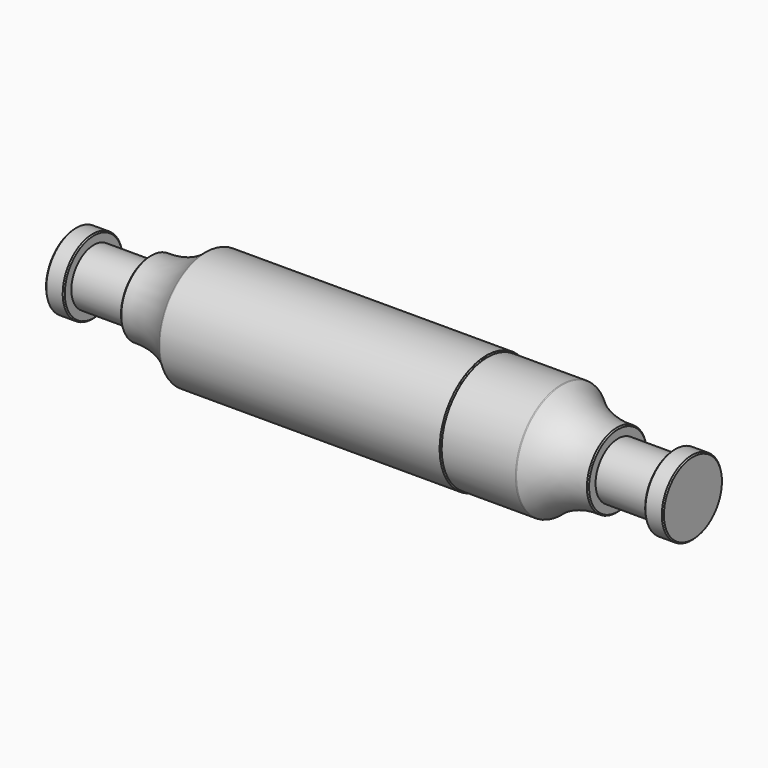
from build123d import *


# Not quite as in the source:
# - a fillet or chamfer that OpenCascade refuses, or shapes differently, is made with other operations: its cross-section is extruded or revolved along the edge and cut away or added


with BuildPart() as f1:
    # F0 (on Front) → F1 (revolve)
    with BuildSketch(Plane.XZ):
        with BuildLine():
            Line((-447.1154779911, 50.8), (-447.1154779911, 0))
            Line((-447.1154779911, 0), (391.0845220089, 0))
            Line((391.0845220089, 0), (391.0845220089, 50.8))
            Line((391.0845220089, 50.8), (365.6845220089, 50.8))
            Line((365.6845220089, 50.8), (365.6845220089, 38.1))
            Line((365.6845220089, 38.1), (289.4845220089, 38.1))
            Line((289.4845220089, 38.1), (289.4845220089, 50.8))
            ThreePointArc((289.4845220089, 50.8), (248.5849137461, 56.3889737285), (213.2845220089, 77.7875))
            Line((213.2845220089, 77.7875), (111.6845220089, 77.7875))
            Line((111.6845220089, 77.7875), (111.6845220089, 79.375))
            Line((111.6845220089, 79.375), (-269.3154779911, 79.375))
            ThreePointArc((-269.3154779911, 79.375), (-304.4294339656, 57.1247159319), (-345.5154779911, 50.8))
            Line((-345.5154779911, 50.8), (-345.5154779911, 38.1))
            Line((-345.5154779911, 38.1), (-421.7154779911, 38.1))
            Line((-421.7154779911, 38.1), (-421.7154779911, 50.8))
            Line((-421.7154779911, 50.8), (-447.1154779911, 50.8))
        make_face()
    revolve(axis=Axis((-28.0154779911, 0, 0), (1, 0, 0)))

    # F2: chamfer of 1.5875 on 8 edges, made by hand

    # F2_s1 → F2_t2 (revolve, cut)
    with BuildSketch(Plane.XZ):
        Polygon((-445.5279779911, 50.8), (-447.1154779911, 49.2125), (-447.1154779911, 50.8), align=None)
    revolve(axis=Axis((-447.1154779911, 0, 0), (1, 0, 0)), mode=Mode.SUBTRACT)

    # F2_s3 → F2_t4 (revolve, cut)
    with BuildSketch(Plane.XZ):
        Polygon((-421.7154779911, 49.2125), (-423.3029779911, 50.8), (-421.7154779911, 50.8), align=None)
    revolve(axis=Axis((-421.7154779911, 0, 0), (1, 0, 0)), mode=Mode.SUBTRACT)

    # F2_s5 → F2_t6 (revolve, cut)
    with BuildSketch(Plane.XZ):
        with BuildLine():
            Line((-343.8691410317, 50.7255652721), (-345.5154779911, 49.1391559736))
            Line((-345.5154779911, 49.1391559736), (-345.5154779911, 50.8))
            ThreePointArc((-345.5154779911, 50.8), (-344.6706324334, 50.7584599548), (-343.8691410317, 50.7255652721))
        make_face()
    revolve(axis=Axis((-345.5154779911, 0, 0), (1, 0, 0)), mode=Mode.SUBTRACT)

    # F2_s7 → F2_t8 (revolve, cut)
    with BuildSketch(Plane.XZ):
        Polygon((391.0845220089, 49.2125), (389.4970220089, 50.8), (391.0845220089, 50.8), align=None)
    revolve(axis=Axis((391.0845220089, 0, 0), (1, 0, 0)), mode=Mode.SUBTRACT)

    # F2_s9 → F2_t10 (revolve, cut)
    with BuildSketch(Plane.XZ):
        Polygon((367.2720220089, 50.8), (365.6845220089, 49.2125), (365.6845220089, 50.8), align=None)
    revolve(axis=Axis((365.6845220089, 0, 0), (1, 0, 0)), mode=Mode.SUBTRACT)

    # F2_s11 → F2_t12 (revolve, cut)
    with BuildSketch(Plane.XZ):
        with BuildLine():
            Line((289.4845220089, 49.1134387616), (287.8140491072, 50.6987689315))
            ThreePointArc((287.8140491072, 50.6987689315), (288.6278622062, 50.7446363641), (289.4845220089, 50.8))
            Line((289.4845220089, 50.8), (289.4845220089, 49.1134387616))
        make_face()
    revolve(axis=Axis((289.4845220089, 0, 0), (1, 0, 0)), mode=Mode.SUBTRACT)

    # F2_s13 → F2_t14 (revolve, cut)
    with BuildSketch(Plane.XZ):
        with BuildLine():
            Line((213.7373414064, 77.3686138432), (212.6628657503, 77.7875))
            Line((212.6628657503, 77.7875), (213.2845220089, 77.7875))
            ThreePointArc((213.2845220089, 77.7875), (213.5323086027, 77.5576500764), (213.7373414064, 77.3686138432))
        make_face()
    revolve(axis=Axis((213.2845220089, 0, 0), (1, 0, 0)), mode=Mode.SUBTRACT)

    # F2_s15 → F2_t16 (revolve, cut)
    with BuildSketch(Plane.XZ):
        with BuildLine():
            Line((-269.7732330498, 78.9331655442), (-268.6743214469, 79.375))
            Line((-268.6743214469, 79.375), (-269.3154779911, 79.375))
            ThreePointArc((-269.3154779911, 79.375), (-269.5651837952, 79.1332927093), (-269.7732330498, 78.9331655442))
        make_face()
    revolve(axis=Axis((-269.3154779911, 0, 0), (1, 0, 0)), mode=Mode.SUBTRACT)

    # F3: chamfer of 0.762 on 4 edges, made by hand

    # F3_s1 → F3_t2 (revolve)
    with BuildSketch(Plane.XZ):
        Polygon((111.6845220089, 78.5495), (112.4465220089, 77.7875), (111.6845220089, 77.7875), align=None)
    revolve(axis=Axis((111.6845220089, 0, 0), (1, 0, 0)))

    # F3_s3 → F3_t4 (revolve, cut)
    with BuildSketch(Plane.XZ):
        Polygon((110.9225220089, 79.375), (111.6845220089, 78.613), (111.6845220089, 79.375), align=None)
    revolve(axis=Axis((111.6845220089, 0, 0), (1, 0, 0)), mode=Mode.SUBTRACT)

    # F3_s5 → F3_t6 (revolve, cut)
    with BuildSketch(Plane.XZ):
        Polygon((212.5195839157, 77.7875), (212.7963616249, 77.7354564069), (212.6628657503, 77.7875), align=None)
    revolve(axis=Axis((212.6628657503, 0, 0), (1, 0, 0)), mode=Mode.SUBTRACT)


solid = f1.part
